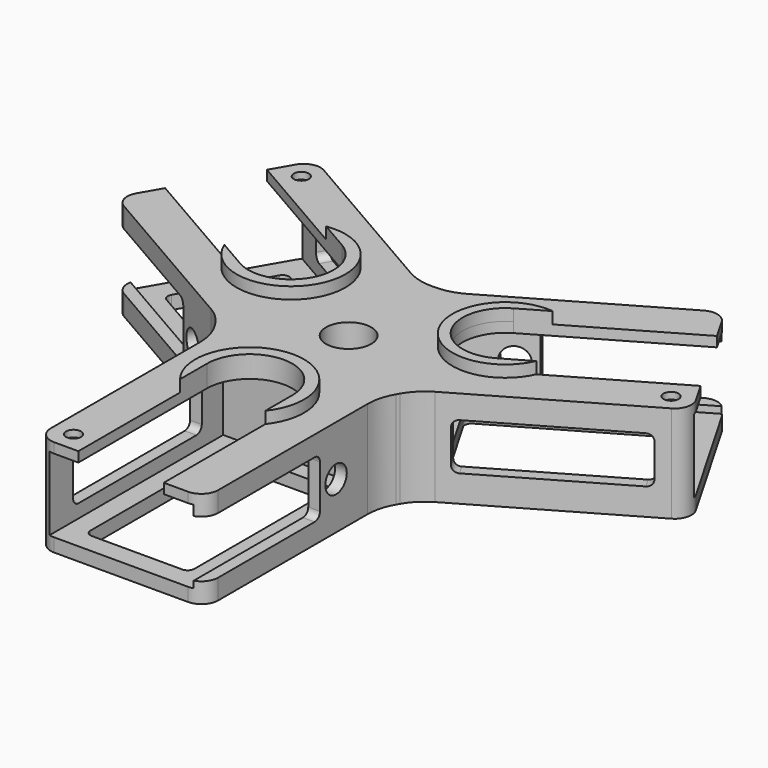
from build123d import *

# Parameters (mm, degrees)
F0_R            = 3.1
F0_R_2          = 12.75
F0_W            = 43
F0_H            = 65
F1_DEPTH        = 4
F2_DEPTH        = 25
F3_START        = 22
F3_DEPTH        = 3
F4_START        = 12.2
F4_DEPTH        = 23.9
F6_DEPTH        = 13.4
F7_DEPTH        = 3.5
F8_W            = 31
F8_H            = 54
F9_DEPTH        = 17
F10_W           = 43
F10_H           = 17
F10_R           = 4
F13_DEPTH       = 25
F11_W           = 43
F11_H           = 17
F11_R           = 4
F14_DEPTH       = 25
F12_W           = 43
F12_H           = 17
F12_R           = 4
F15_DEPTH       = 25
F16_W           = 48
F16_H           = 14
F19_DEPTH       = 25
F17_W           = 48
F17_H           = 14
F20_DEPTH       = 25
F18_W           = 48
F18_H           = 14
F21_DEPTH       = 25
F22_R           = 16
F23_T1_DEPTH    = 31
F23_T3_DEPTH    = 31
F23_T5_DEPTH    = 54
F24_D           = 2.1
F24_DEPTH       = 6
F24_CBORE_D     = 4.5
F24_CBORE_DEPTH = 2
F24_TIP         = 0.63090365
F25_D           = 6.2
F25_DEPTH       = 30
F25_CBORE_D     = 13.5
F25_CBORE_DEPTH = 20
F25_TIP         = 1.862667919
F26_R           = 2


# Not quite as in the source:
# - a fillet or chamfer that OpenCascade refuses, or shapes differently, is made with other operations: its cross-section is extruded or revolved along the edge and cut away or added


with BuildPart() as f1:
    # F0 (on Top) → F1 (new body)
    with BuildSketch(Plane.XY):
        Polygon((21.5, -19.9504172281), (21.5, -84.9504172281), (25, -84.9504172281), (25, -19.9504172281), (29.7775681357, -11.6754264805), (86.0692193817, 20.8245735195), (84.3192193817, 23.8556624327), (28.0275681357, -8.6443375673), (6.5275681357, 28.5947547954), (62.8192193817, 61.0947547954), (61.0692193817, 64.1258437087), (4.7775681357, 31.6258437087), (-4.7775681357, 31.6258437087), (-61.0692193817, 64.1258437087), (-62.8192193817, 61.0947547954), (-6.5275681357, 28.5947547954), (-28.0275681357, -8.6443375673), (-84.3192193817, 23.8556624327), (-86.0692193817, 20.8245735195), (-29.7775681357, -11.6754264805), (-25, -19.9504172281), (-25, -84.9504172281), (-21.5, -84.9504172281), (-21.5, -19.9504172281), align=None)
        Circle(F0_R, mode=Mode.SUBTRACT)
        Polygon((-62.8192193817, 61.0947547954), (-84.3192193817, 23.8556624327), (-28.0275681357, -8.6443375673), (-6.5275681357, 28.5947547954), align=None)
        with Locations((-32, 18.4752086141)):
            Circle(F0_R_2, mode=Mode.SUBTRACT)
        Polygon((28.0275681357, -8.6443375673), (84.3192193817, 23.8556624327), (62.8192193817, 61.0947547954), (6.5275681357, 28.5947547954), align=None)
        with Locations((32, 18.4752086141)):
            Circle(F0_R_2, mode=Mode.SUBTRACT)
        with Locations((0, -52.4504172281)):
            Rectangle(F0_W, F0_H)
        with Locations((0, -36.9504172281)):
            Circle(F0_R_2, mode=Mode.SUBTRACT)
        with Locations((-32, 18.4752086141)):
            Circle(F0_R_2)
        with Locations((32, 18.4752086141)):
            Circle(F0_R_2)
        with Locations((0, -36.9504172281)):
            Circle(F0_R_2)
    extrude(amount=-F1_DEPTH)

    # F0 (on Top) → F2 (join)
    with BuildSketch(Plane.XY):
        Polygon((21.5, -19.9504172281), (21.5, -84.9504172281), (25, -84.9504172281), (25, -19.9504172281), (29.7775681357, -11.6754264805), (86.0692193817, 20.8245735195), (84.3192193817, 23.8556624327), (28.0275681357, -8.6443375673), (6.5275681357, 28.5947547954), (62.8192193817, 61.0947547954), (61.0692193817, 64.1258437087), (4.7775681357, 31.6258437087), (-4.7775681357, 31.6258437087), (-61.0692193817, 64.1258437087), (-62.8192193817, 61.0947547954), (-6.5275681357, 28.5947547954), (-28.0275681357, -8.6443375673), (-84.3192193817, 23.8556624327), (-86.0692193817, 20.8245735195), (-29.7775681357, -11.6754264805), (-25, -19.9504172281), (-25, -84.9504172281), (-21.5, -84.9504172281), (-21.5, -19.9504172281), align=None)
        Circle(F0_R, mode=Mode.SUBTRACT)
    extrude(amount=F2_DEPTH)

    # F0 (on Top) → F3 (join)
    with BuildSketch(Plane.XY.offset(F3_START)):
        with Locations((0, -52.4504172281)):
            Rectangle(F0_W, F0_H)
        with Locations((0, -36.9504172281)):
            Circle(F0_R_2, mode=Mode.SUBTRACT)
        Polygon((-62.8192193817, 61.0947547954), (-84.3192193817, 23.8556624327), (-28.0275681357, -8.6443375673), (-6.5275681357, 28.5947547954), align=None)
        with Locations((-32, 18.4752086141)):
            Circle(F0_R_2, mode=Mode.SUBTRACT)
        Polygon((28.0275681357, -8.6443375673), (84.3192193817, 23.8556624327), (62.8192193817, 61.0947547954), (6.5275681357, 28.5947547954), align=None)
        with Locations((32, 18.4752086141)):
            Circle(F0_R_2, mode=Mode.SUBTRACT)
    extrude(amount=F3_DEPTH)

    # F0 (on Top) → F4 (cut)
    with BuildSketch(Plane.XY.offset(F4_START)):
        with Locations((32, 18.4752086141)):
            Circle(F0_R_2)
        with Locations((-32, 18.4752086141)):
            Circle(F0_R_2)
        with Locations((0, -36.9504172281)):
            Circle(F0_R_2)
    extrude(amount=F4_DEPTH, mode=Mode.SUBTRACT)

    # F5 (on face) → F6 (cut)
    with BuildSketch(Plane.XY.offset(25)):
        with BuildLine():
            Line((-67.1942193817, 53.5170325123), (-79.9442193817, 31.4333847158))
            Line((-79.9442193817, 31.4333847158), (-47.0999641833, 12.4707451357))
            Line((-47.0999641833, 12.4707451357), (-38.375, 7.4333847158))
            ThreePointArc((-38.375, 7.4333847158), (-43.0418238983, 24.8502086141), (-25.625, 29.5170325123))
            Line((-25.625, 29.5170325123), (-34.3499641833, 34.5543929322))
            Line((-34.3499641833, 34.5543929322), (-67.1942193817, 53.5170325123))
        make_face()
        with BuildLine():
            Line((46.382808689, 12.056695218), (79.9442193817, 31.4333847158))
            Line((79.9442193817, 31.4333847158), (67.1942193817, 53.5170325123))
            Line((67.1942193817, 53.5170325123), (33.632808689, 34.1403430145))
            Line((33.632808689, 34.1403430145), (25.625, 29.5170325123))
            ThreePointArc((25.625, 29.5170325123), (38.375, 29.5170325123), (44.75, 18.4752086141))
            ThreePointArc((44.75, 18.4752086141), (43.0418238983, 12.1002086141), (38.375, 7.4333847158))
            Line((38.375, 7.4333847158), (46.382808689, 12.056695218))
        make_face()
        with BuildLine():
            Line((12.75, -47.0251380679), (12.75, -36.9504172281))
            ThreePointArc((12.75, -36.9504172281), (0, -49.7004172281), (-12.75, -36.9504172281))
            Line((-12.75, -36.9504172281), (-12.75, -47.0251380679))
            Line((-12.75, -47.0251380679), (-12.75, -84.9504172281))
            Line((-12.75, -84.9504172281), (12.75, -84.9504172281))
            Line((12.75, -84.9504172281), (12.75, -47.0251380679))
        make_face()
    extrude(amount=-F6_DEPTH, mode=Mode.SUBTRACT)

    # F5 (on face) → F7 (join)
    with BuildSketch(Plane.XY.offset(25)):
        with BuildLine():
            Line((-38.375, 7.4333847158), (-47.0999641833, 12.4707451357))
            ThreePointArc((-47.0999641833, 12.4707451357), (-17.9270871885, 10.3502086141), (-34.3499641833, 34.5543929322))
            Line((-34.3499641833, 34.5543929322), (-25.625, 29.5170325123))
            ThreePointArc((-25.625, 29.5170325123), (-20.9581761017, 24.8502086141), (-19.25, 18.4752086141))
            ThreePointArc((-19.25, 18.4752086141), (-25.625, 7.4333847158), (-38.375, 7.4333847158))
        make_face()
        with BuildLine():
            ThreePointArc((33.632808689, 34.1403430145), (18.3600998904, 10.6002086141), (46.382808689, 12.056695218))
            Line((46.382808689, 12.056695218), (38.375, 7.4333847158))
            ThreePointArc((38.375, 7.4333847158), (20.9581761017, 12.1002086141), (25.625, 29.5170325123))
            Line((25.625, 29.5170325123), (33.632808689, 34.1403430145))
        make_face()
        with BuildLine():
            ThreePointArc((-12.75, -36.9504172281), (0, -24.2004172281), (12.75, -36.9504172281))
            Line((12.75, -36.9504172281), (12.75, -47.0251380679))
            ThreePointArc((12.75, -47.0251380679), (0, -20.7004172281), (-12.75, -47.0251380679))
            Line((-12.75, -47.0251380679), (-12.75, -36.9504172281))
        make_face()
    extrude(amount=F7_DEPTH)

    # F8 (on face) → F9 (cut)
    with BuildSketch(Plane(origin=(0, 0, -4), x_dir=(1, 0, 0), z_dir=(0, 0, -1))):
        Polygon((29.3576951546, 0.9481851446), (13.8576951546, -25.8986023727), (60.6230669589, -52.8986023727), (76.1230669589, -26.0518148554), align=None)
        with Locations((0, 51.9504172281)):
            Rectangle(F8_W, F8_H)
        Polygon((-13.8576951546, -25.8986023727), (-29.3576951546, 0.9481851446), (-76.1230669589, -26.0518148554), (-60.6230669589, -52.8986023727), align=None)
    extrude(amount=-F9_DEPTH, mode=Mode.SUBTRACT)

    # F10 (on face) → F13 (cut)
    with BuildSketch(Plane(origin=(-12.5, 21.6506350946, 0), x_dir=(-0.8660254038, -0.5, 0), z_dir=(-0.5, 0.8660254038, 0))):
        with Locations((-63.4504172281, 10.5)):
            Rectangle(F10_W, F10_H)
        with Locations((-35.9504172281, 10)):
            Circle(F10_R)
    extrude(amount=-F13_DEPTH, mode=Mode.SUBTRACT)

    # F11 (on face) → F14 (cut)
    with BuildSketch(Plane(origin=(-12.5, -21.6506350946, 0), x_dir=(0.8660254038, -0.5, 0), z_dir=(-0.5, -0.8660254038, 0))):
        with Locations((-63.4504172281, 10.5)):
            Rectangle(F11_W, F11_H)
        with Locations((-35.9504172281, 10)):
            Circle(F11_R)
    extrude(amount=-F14_DEPTH, mode=Mode.SUBTRACT)

    # F12 (on face) → F15 (cut)
    with BuildSketch(Plane.YZ.offset(25)):
        with Locations((-63.4504172281, 10.5)):
            Rectangle(F12_W, F12_H)
        with Locations((-35.9504172281, 10)):
            Circle(F12_R)
    extrude(amount=-F15_DEPTH, mode=Mode.SUBTRACT)

    # F16 (on face) → F19 (cut)
    with BuildSketch(Plane(origin=(-25, 0, 0), x_dir=(0, -1, 0), z_dir=(-1, 0, 0))):
        with Locations((51.9504172281, 11)):
            Rectangle(F16_W, F16_H)
    extrude(amount=-F19_DEPTH, mode=Mode.SUBTRACT)

    # F17 (on face) → F20 (cut)
    with BuildSketch(Plane(origin=(12.5, -21.6506350946, 0), x_dir=(0.8660254038, 0.5, 0), z_dir=(0.5, -0.8660254038, 0))):
        with Locations((51.9504172281, 11)):
            Rectangle(F17_W, F17_H)
    extrude(amount=-F20_DEPTH, mode=Mode.SUBTRACT)

    # F18 (on face) → F21 (cut)
    with BuildSketch(Plane(origin=(12.5, 21.6506350946, 0), x_dir=(-0.8660254038, 0.5, 0), z_dir=(0.5, 0.8660254038, 0))):
        with Locations((51.9504172281, 11)):
            Rectangle(F18_W, F18_H)
    extrude(amount=-F21_DEPTH, mode=Mode.SUBTRACT)

    # F22
    f22_edges = [f1.edges().sort_by_distance(p)[0] for p in [
        (29.777568, -11.675426, 10.5),
        (25, -19.950417, 10.5),
        (-4.777568, 31.625844, 10.5),
        (4.777568, 31.625844, 10.5),
        (-25, -19.950417, 10.5),
        (-29.777568, -11.675426, 10.5),
    ]]
    fillet(f22_edges, radius=F22_R)

    # F23: fillet of radius 5 on 9 edges, made by hand

    # F23_s2 → F23_t1 (cut)
    with BuildSketch(Plane.XY.offset(6.5)):
        with BuildLine():
            ThreePointArc((-81.7390923627, 18.3245735195), (-84.0687214942, 21.3606053129), (-83.5692193817, 25.1547005384))
            Line((-83.5692193817, 25.1547005384), (-86.0692193817, 20.8245735195))
            Line((-86.0692193817, 20.8245735195), (-81.7390923627, 18.3245735195))
        make_face()
        with BuildLine():
            ThreePointArc((25, -79.9504172281), (23.5355339059, -83.4859511341), (20, -84.9504172281))
            Line((20, -84.9504172281), (25, -84.9504172281))
            Line((25, -84.9504172281), (25, -79.9504172281))
        make_face()
        with BuildLine():
            ThreePointArc((56.7390923627, 61.6258437087), (60.5331875882, 62.1253458212), (63.5692193817, 59.7957166898))
            Line((63.5692193817, 59.7957166898), (61.0692193817, 64.1258437087))
            Line((61.0692193817, 64.1258437087), (56.7390923627, 61.6258437087))
        make_face()
    extrude(amount=F23_T1_DEPTH, mode=Mode.SUBTRACT)

    # F23_s4 → F23_t3 (cut)
    with BuildSketch(Plane.XY.offset(-16.5)):
        with BuildLine():
            ThreePointArc((-81.7390923627, 18.3245735195), (-84.0687214942, 21.3606053129), (-83.5692193817, 25.1547005384))
            Line((-83.5692193817, 25.1547005384), (-86.0692193817, 20.8245735195))
            Line((-86.0692193817, 20.8245735195), (-81.7390923627, 18.3245735195))
        make_face()
        with BuildLine():
            ThreePointArc((20, -84.9504172281), (23.5355339059, -83.4859511341), (25, -79.9504172281))
            Line((25, -79.9504172281), (25, -84.9504172281))
            Line((25, -84.9504172281), (20, -84.9504172281))
        make_face()
        with BuildLine():
            ThreePointArc((63.5692193817, 59.7957166898), (60.5331875882, 62.1253458212), (56.7390923627, 61.6258437087))
            Line((56.7390923627, 61.6258437087), (61.0692193817, 64.1258437087))
            Line((61.0692193817, 64.1258437087), (63.5692193817, 59.7957166898))
        make_face()
    extrude(amount=F23_T3_DEPTH, mode=Mode.SUBTRACT)

    # F23_s6 → F23_t5 (cut)
    with BuildSketch(Plane.XY.offset(-16.5)):
        with BuildLine():
            ThreePointArc((-63.5692193817, 59.7957166898), (-60.5331875882, 62.1253458212), (-56.7390923627, 61.6258437087))
            Line((-56.7390923627, 61.6258437087), (-61.0692193817, 64.1258437087))
            Line((-61.0692193817, 64.1258437087), (-63.5692193817, 59.7957166898))
        make_face()
        with BuildLine():
            ThreePointArc((-25, -79.9504172281), (-23.5355339059, -83.4859511341), (-20, -84.9504172281))
            Line((-20, -84.9504172281), (-25, -84.9504172281))
            Line((-25, -84.9504172281), (-25, -79.9504172281))
        make_face()
        with BuildLine():
            ThreePointArc((81.7390923627, 18.3245735195), (84.0687214942, 21.3606053129), (83.5692193817, 25.1547005384))
            Line((83.5692193817, 25.1547005384), (86.0692193817, 20.8245735195))
            Line((86.0692193817, 20.8245735195), (81.7390923627, 18.3245735195))
        make_face()
    extrude(amount=F23_T5_DEPTH, mode=Mode.SUBTRACT)

    # F24
    with Locations(Plane.XY.offset(25)):
        with Locations((-19, -78.9504172281), (77.8730669589, 23.0207259422), (-58.8730669589, 55.929691286)):
            CounterBoreHole(F24_D / 2, F24_CBORE_D / 2, F24_CBORE_DEPTH, depth=F24_DEPTH)
            with Locations((0, 0, -(F24_DEPTH + F24_TIP / 2))):  # 118° drill point
                Cone(0, F24_D / 2, F24_TIP, mode=Mode.SUBTRACT)

    # F25
    with Locations(Plane.XY.offset(25)):
        with Locations((0, 0)):
            CounterBoreHole(F25_D / 2, F25_CBORE_D / 2, F25_CBORE_DEPTH, depth=F25_DEPTH)
            with Locations((0, 0, -(F25_DEPTH + F25_TIP / 2))):  # 118° drill point
                Cone(0, F25_D / 2, F25_TIP, mode=Mode.SUBTRACT)

    # F26
    f26_edges = [f1.edges().sort_by_distance(p)[0] for p in [
        (-12.580771, 34.110299, 18),
        (-54.149991, 58.110299, 18),
        (-54.149991, 58.110299, 4),
        (-12.580771, 34.110299, 4),
        (-23.25, -27.950417, 4),
        (-23.25, -75.950417, 4),
        (-23.25, -75.950417, 18),
        (-23.25, -27.950417, 18),
        (23.25, -41.950417, 19),
        (23.25, -41.950417, 2),
        (35.830771, -6.159882, 4),
        (35.830771, -6.159882, 18),
        (77.399991, 17.840118, 4),
        (77.399991, 17.840118, 18),
        (24.705127, 41.110299, 19),
        (24.705127, 41.110299, 2),
        (-47.955127, 0.840118, 19),
        (-47.955127, 0.840118, 2),
        (-60.623067, 52.898602, -2),
        (-76.123067, 26.051815, -2),
        (-29.357695, -0.948185, -2),
        (-13.857695, 25.898602, -2),
        (13.857695, 25.898602, -2),
        (60.623067, 52.898602, -2),
        (15.5, -78.950417, -2),
        (-15.5, -78.950417, -2),
        (29.357695, -0.948185, -2),
        (76.123067, 26.051815, -2),
        (15.5, -24.950417, -2),
        (-15.5, -24.950417, -2),
    ]]
    fillet(f26_edges, radius=F26_R)


solid = f1.part
